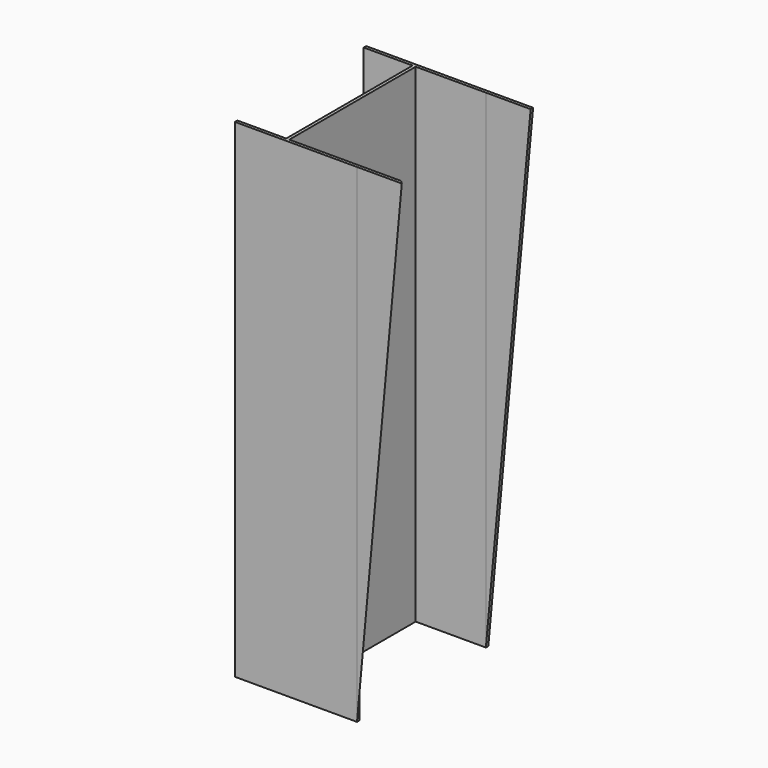
from build123d import *

# Parameters (mm, degrees)
F1_DEPTH = 3000
F3_DEPTH = 19
F5_DEPTH = 19
F6_SIZE  = 18.99999


# Not quite as in the source:
# - a fillet or chamfer is up to 0.001 mm smaller than in the source, because OpenCascade refuses the exact size


with BuildPart() as f1:
    # F0 (on Top) → F1 (new body)
    with BuildSketch(Plane.XY):
        Polygon((0, 19), (0, 0), (750, 0), (750, 19), (319, 19), (319, 989), (750, 989), (750, 1008), (0, 1008), (0, 989), (300, 989), (300, 19), align=None)
    extrude(amount=F1_DEPTH)


with BuildPart() as f3:
    # F2 (on face) → F3 (new body)
    with BuildSketch(Plane.XZ):
        Polygon((1025, 3000), (750, 3000), (750, 0), align=None)
    extrude(amount=-F3_DEPTH)

    # F6 (size 19 in the source; OpenCascade refuses exactly that, so slightly less here)
    f6_edges = [f3.edges().sort_by_distance(p)[0] for p in [
        (887.5, 19, 1500),
    ]]
    chamfer(f6_edges, length=F6_SIZE)


with BuildPart() as f5:
    # F4 (on face) → F5 (new body)
    with BuildSketch(Plane(origin=(0, 1008, 0), x_dir=(-1, 0, 0), z_dir=(0, 1, 0))):
        Polygon((-750, 0), (-750, 3000), (-1025, 3000), align=None)
    extrude(amount=-F5_DEPTH)


solid = Compound([f1.part, f3.part, f5.part])
